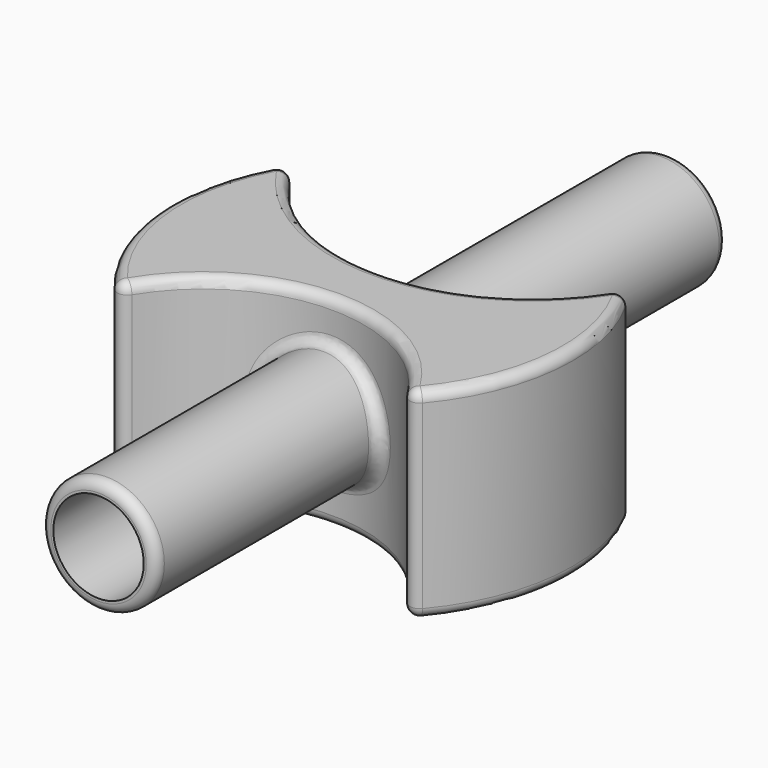
from build123d import *

# Parameters (mm, degrees)
F1_DEPTH      = 10
F2_R          = 5.75
F3_DEPTH      = 34
F3_DEPTH_BACK = 37
F4_R          = 4.5
F5_DEPTH      = 71.0010001
F6_R          = 1


with BuildPart() as f1:
    # F0 (on Top) → F1 (new body, symmetric)
    with BuildSketch(Plane.XY):
        with BuildLine():
            ThreePointArc((14.3525223553, -13.9285714286), (18.5344334565, -7.5149701561), (20, 0))
            ThreePointArc((20, 0), (19.1623928859, 5.7273640434), (16.7197301115, 10.975))
            ThreePointArc((16.7197301115, 10.975), (0, 1), (-16.7197301115, 10.975))
            ThreePointArc((-16.7197301115, 10.975), (-19.9102532835, -1.8925681457), (-14.3525223553, -13.9285714286))
            ThreePointArc((-14.3525223553, -13.9285714286), (0, -5), (14.3525223553, -13.9285714286))
        make_face()
    extrude(amount=F1_DEPTH, both=True)

    # F2 (on Front) → F3 (join, two sides)
    with BuildSketch(Plane.XZ) as f3_sk:
        Circle(F2_R)
    extrude(amount=F3_DEPTH)
    extrude(f3_sk.sketch, amount=-F3_DEPTH_BACK)

    # F4 (on face) → F5 (cut, through all)
    with BuildSketch(Plane.XZ.offset(34)):
        Circle(F4_R)
    extrude(amount=-F5_DEPTH, mode=Mode.SUBTRACT)

    # F6
    f6_edges = [f1.edges().sort_by_distance(p)[0] for p in [
        (-19.910253, -1.892568, -10),
        (0, -5, -10),
        (19.910253, -1.892568, -10),
        (0, 1, -10),
        (-19.910253, -1.892568, 10),
        (0, -5, 10),
        (19.910253, -1.892568, 10),
        (0, 1, 10),
        (-14.352522, -13.928571, 0),
        (14.352522, -13.928571, 0),
        (16.71973, 10.975, 0),
        (-16.71973, 10.975, 0),
        (-5.75, -34, 0),
        (-5.75, 37, 0),
        (-5.75, 1.890955, 0),
        (-5.749998, -6.068908, 0.004262),
    ]]
    fillet(f6_edges, radius=F6_R)


solid = f1.part
